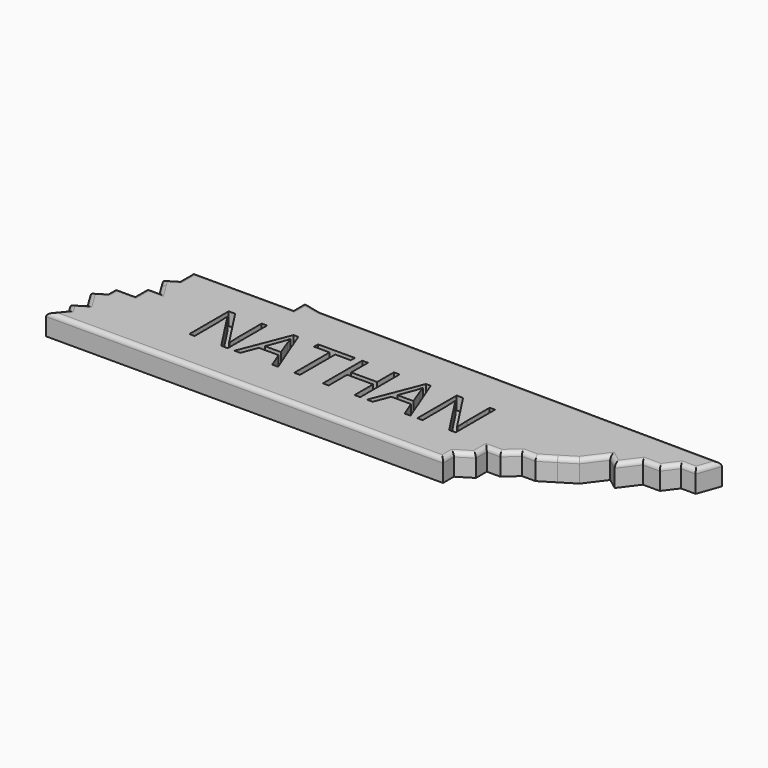
from build123d import *

# Parameters (mm, degrees)
F1_DEPTH     = 5
F2_R         = 1
F3_TEXT_SIZE = 15.830593313
F4_DEPTH     = 3


# Not quite as in the source:
# - Text() gives the source's letters only with a copy of the font that has no kerning and outlines rounded to 1/6400 em; it was checked with that copy


with BuildPart() as f1:
    # F0 (on Top) → F1 (new body)
    with BuildSketch(Plane.XY):
        Polygon((61.2789727747, 9.9089415744), (64.6688789129, 9.9089415744), (66.517367959, 15.1401581243), (-26.3369232416, 15.9064587206), (-30.7698696852, 16.9495046139), (-30.7698696852, 13.5596040636), (-53.7168905139, 13.5596040636), (-53.7168905139, 9.492722097), (-56.3245043159, 7.888037755), (-55.0240552017, 5.7748065294), (-53.7168905139, 3.6506624892), (-56.3245043159, 3.6506624892), (-56.3245043159, 0), (-60.7262012062, 0), (-60.7262012062, -2.4302292567), (-63.3450093178, -4.0418024), (-60.7262012062, -8.2973684311), (-63.3450093178, -9.9089415744), (-62.0612613857, -11.995033361), (-64.6688789129, -15.1241719723), (26.5976823866, -15.1241719723), (26.5976823866, -11.995033361), (29.9875866622, -9.9089415744), (29.9875866622, -6.7798020318), (33.1167243421, -6.7798020318), (35.9851010144, -4.1721854359), (39.114240557, -4.1721854359), (42.5041429698, -2.0860927179), (45.8940459066, 0), (49.304804446, 4.5476781371), (51.891554147, 2.6076158974), (55.0206936896, 6.7798020318), (58.9321181178, 6.7798020318), align=None)
    extrude(amount=F1_DEPTH)

    # F2
    f2_edges = [f1.edges().sort_by_distance(p)[0] for p in [
        (-28.553396, 16.427982, 5),
        (-42.24338, 13.559604, 5),
        (-53.716891, 11.526163, 5),
        (-55.020697, 8.69038, 5),
        (-55.020697, 5.76935, 5),
        (-30.76987, 15.254554, 5),
        (20.090222, 15.523308, 5),
        (-55.020697, 3.650662, 5),
        (-56.324504, 1.825331, 5),
        (-58.525353, 0, 5),
        (-60.726201, -1.215115, 5),
        (-62.035605, -3.236016, 5),
        (-62.035605, -6.169585, 5),
        (-62.035605, -9.103155, 5),
        (-62.703135, -10.951987, 5),
        (-63.36507, -13.559603, 5),
        (-19.035598, -15.124172, 5),
        (26.597682, -13.559603, 5),
        (28.292635, -10.951987, 5),
        (29.987587, -8.344372, 5),
        (31.552156, -6.779802, 5),
        (34.550913, -5.475994, 5),
        (37.549671, -4.172185, 5),
        (44.199094, -1.043046, 5),
        (40.809192, -3.129139, 5),
        (47.599425, 2.273839, 5),
        (50.598179, 3.577647, 5),
        (53.456124, 4.693709, 5),
        (56.976406, 6.779802, 5),
        (60.105545, 8.344372, 5),
        (62.973926, 9.908942, 5),
        (65.593123, 12.52455, 5),
    ]]
    fillet(f2_edges, radius=F2_R)

    # F3 (on face) → F4 (cut)
    with BuildSketch(Plane.XY.offset(5)):
        with Locations((-40.7072380185, -5.8343410492)):
            Text('NATHAN', F3_TEXT_SIZE, font='Open Sans', text_align=(TextAlign.LEFT, TextAlign.BOTTOM))
    extrude(amount=-F4_DEPTH, mode=Mode.SUBTRACT)


solid = f1.part
